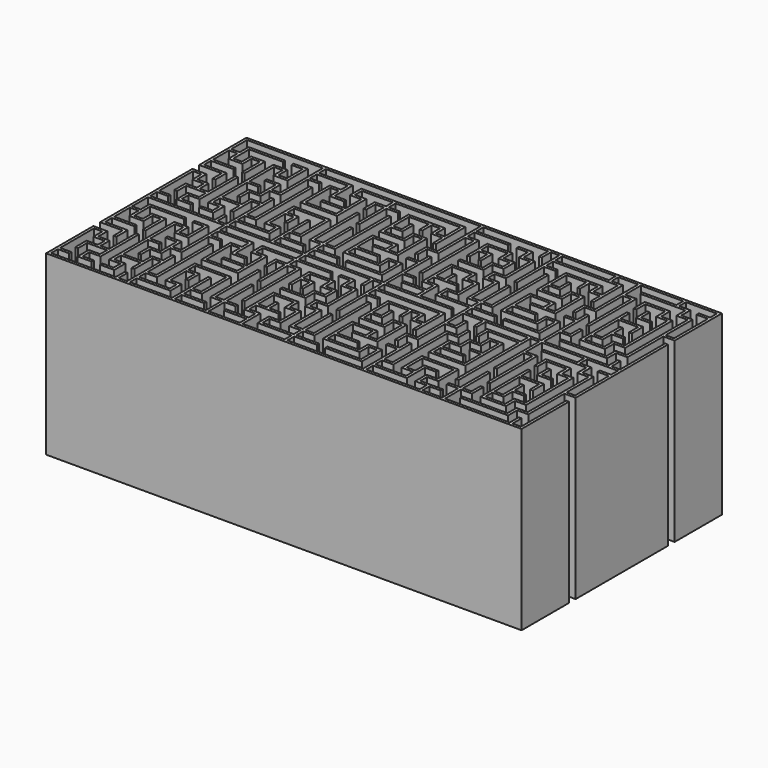
from build123d import *

# Parameters (mm, degrees)
F0_W     = 1.5875
F0_H     = 0.396875
F0_W_2   = 4.7625
F1_DEPTH = 25
F0_W_3   = 0.396875
F0_H_2   = 1.5875
F0_W_4   = 3.175
F0_H_3   = 7.9375
F0_W_5   = 10.715625


# Not quite as in the source:
# - a feature of the source that left no trace in its solid (it failed there, or was rolled back) is left out


with BuildPart() as f1:
    # F0 (on Top) → F1 (new body)
    with BuildSketch(Plane.XY):
        Polygon((-25.598351, 8.135938), (-25.598351, 6.151563), (-25.201476, 6.151563), (-25.201476, 7.739063), (-23.613976, 7.739063), (-23.613976, 9.326563), (-22.423351, 9.326563), (-22.423351, 9.723438), (-23.613976, 9.723438), (-23.613976, 11.310938), (-25.598351, 11.310938), (-25.598351, 10.914063), (-24.010851, 10.914063), (-24.010851, 8.135938), align=None)
        Polygon((-22.423351, 9.723438), (-22.423351, 9.326563), (-22.026476, 9.326563), (-22.026476, 14.089063), (-22.026476, 14.485938), (-22.026476, 15.676563), (-22.026476, 16.073438), (-22.026476, 17.264063), (-22.026476, 17.660938), (-22.423351, 17.660938), (-22.423351, 17.264063), align=None)
        with Locations((-21.232726, 14.2875005)):
            Rectangle(F0_W, F0_H)
        Polygon((-33.138976, 17.264063), (-22.423351, 17.264063), (-22.423351, 17.660938), (-33.535851, 17.660938), (-33.535851, 9.326563), (-30.360851, 9.326563), (-30.360851, 7.739063), (-29.963976, 7.739063), (-29.963976, 9.723438), (-33.138976, 9.723438), (-33.138976, 10.914063), (-29.963976, 10.914063), (-29.963976, 11.310938), (-33.138976, 11.310938), (-33.138976, 14.089063), (-31.948351, 14.089063), (-31.948351, 12.501563), (-29.963976, 12.501563), (-29.963976, 14.089063), (-28.773351, 14.089063), (-28.773351, 10.914063), (-28.376476, 10.914063), (-28.376476, 14.485938), (-30.360851, 14.485938), (-30.360851, 12.898438), (-31.551476, 12.898438), (-31.551476, 15.676563), (-26.788976, 15.676563), (-26.788976, 16.073438), (-31.948351, 16.073438), (-31.948351, 14.485938), (-33.138976, 14.485938), align=None)
        Polygon((-22.026476, 16.073438), (-22.026476, 15.676563), (-17.660851, 15.676563), (-17.660851, 14.485938), (-19.248351, 14.485938), (-19.248351, 9.326563), (-14.088976, 9.326563), (-14.088976, 14.485938), (-15.676476, 14.485938), (-15.676476, 15.676563), (-11.310851, 15.676563), (-11.310851, 14.485938), (-12.898351, 14.485938), (-12.898351, 12.501563), (-12.501476, 12.501563), (-12.501476, 14.089063), (-11.310851, 14.089063), (-11.310851, 9.326563), (-10.913976, 9.326563), (-10.913976, 14.089063), (-9.326476, 14.089063), (-9.326476, 14.485938), (-10.913976, 14.485938), (-10.913976, 15.676563), (-1.786023, 15.676563), (-1.786023, 12.898438), (-2.976648, 12.898438), (-2.976648, 14.485938), (-8.135851, 14.485938), (-8.135851, 9.326563), (-4.564148, 9.326563), (-4.564148, 10.914063), (-3.373523, 10.914063), (-3.373523, 6.548438), (-4.564148, 6.548438), (-4.564148, 8.135938), (-8.135851, 8.135938), (-8.135851, 2.976563), (-2.976648, 2.976563), (-2.976648, 4.564063), (-1.786023, 4.564063), (-1.786023, 1.785938), (-6.548351, 1.785938), (-6.548351, 1.389063), (-1.389148, 1.389063), (-1.389148, 4.960938), (-3.373523, 4.960938), (-3.373523, 3.373438), (-7.738976, 3.373438), (-7.738976, 4.564063), (-4.564148, 4.564063), (-4.564148, 4.960938), (-7.738976, 4.960938), (-7.738976, 7.739063), (-4.961023, 7.739063), (-4.961023, 6.548438), (-6.548351, 6.548438), (-6.548351, 6.151563), (-2.976648, 6.151563), (-2.976648, 11.310938), (-4.961023, 11.310938), (-4.961023, 9.723438), (-7.738976, 9.723438), (-7.738976, 10.914063), (-6.151476, 10.914063), (-6.151476, 12.898438), (-6.548351, 12.898438), (-6.548351, 11.310938), (-7.738976, 11.310938), (-7.738976, 14.089063), (-4.961023, 14.089063), (-4.961023, 12.501563), (-4.564148, 12.501563), (-4.564148, 14.089063), (-3.373523, 14.089063), (-3.373523, 12.501563), (-1.786023, 12.501563), (-1.786023, 10.914063), (-1.389148, 10.914063), (-1.389148, 16.073438), (-2.976648, 16.073438), (-3.373523, 16.073438), (-10.913976, 16.073438), (-11.310851, 16.073438), (-16.073351, 16.073438), (-16.073351, 14.089063), (-14.485851, 14.089063), (-14.485851, 11.310938), (-17.660851, 11.310938), (-17.660851, 10.914063), (-14.485851, 10.914063), (-14.485851, 9.723438), (-18.851476, 9.723438), (-18.851476, 14.089063), (-17.660851, 14.089063), (-17.660851, 12.501563), (-15.676476, 12.501563), (-15.676476, 12.898438), (-17.263976, 12.898438), (-17.263976, 16.073438), align=None)
        Polygon((-11.310851, 17.660938), (-22.026476, 17.660938), (-22.026476, 17.264063), (-11.310851, 17.264063), (-10.913976, 17.264063), (-3.373523, 17.264063), (-2.976648, 17.264063), (-0.198523, 17.264063), (-0.198523, 9.723438), (-0.198523, 9.326563), (0.198352, 9.326563), (0.198352, 14.089063), (0.198352, 14.485938), (0.198352, 15.676563), (0.198352, 16.073438), (0.198352, 17.264063), (9.326477, 17.264063), (9.326477, 15.676563), (9.723352, 15.676563), (9.723352, 17.264063), (10.913977, 17.264063), (10.913977, 17.660938), (0.198352, 17.660938), (-0.198523, 17.660938), (-10.913976, 17.660938), align=None)
        Polygon((11.310852, 17.660938), (10.913977, 17.660938), (10.913977, 17.264063), (10.913977, 9.326563), (11.310852, 9.326563), (11.310852, 14.089063), (11.310852, 14.485938), (11.310852, 15.676563), (11.310852, 16.073438), (11.310852, 17.264063), align=None)
        Polygon((22.026477, 17.660938), (11.310852, 17.660938), (11.310852, 17.264063), (18.851477, 17.264063), (18.851477, 16.073438), (11.310852, 16.073438), (11.310852, 15.676563), (20.438977, 15.676563), (20.438977, 12.898438), (19.248352, 12.898438), (19.248352, 14.485938), (14.088977, 14.485938), (14.088977, 9.326563), (17.660852, 9.326563), (17.660852, 10.914063), (18.851477, 10.914063), (18.851477, 6.548438), (17.660852, 6.548438), (17.660852, 8.135938), (14.088977, 8.135938), (14.088977, 2.976563), (19.248352, 2.976563), (19.248352, 4.564063), (20.438977, 4.564063), (20.438977, 1.785938), (15.676477, 1.785938), (15.676477, 1.389063), (20.835852, 1.389063), (20.835852, 4.960938), (18.851477, 4.960938), (18.851477, 3.373438), (14.485852, 3.373438), (14.485852, 4.564063), (17.660852, 4.564063), (17.660852, 4.960938), (14.485852, 4.960938), (14.485852, 7.739063), (17.263977, 7.739063), (17.263977, 6.548438), (15.676477, 6.548438), (15.676477, 6.151563), (19.248352, 6.151563), (19.248352, 11.310938), (17.263977, 11.310938), (17.263977, 9.723438), (14.485852, 9.723438), (14.485852, 10.914063), (16.073352, 10.914063), (16.073352, 12.898438), (15.676477, 12.898438), (15.676477, 11.310938), (14.485852, 11.310938), (14.485852, 14.089063), (17.263977, 14.089063), (17.263977, 12.501563), (17.660852, 12.501563), (17.660852, 14.089063), (18.851477, 14.089063), (18.851477, 12.501563), (20.438977, 12.501563), (20.438977, 10.914063), (20.835852, 10.914063), (20.835852, 16.073438), (19.248352, 16.073438), (19.248352, 17.264063), (22.026477, 17.264063), align=None)
        Polygon((-0.198523, 9.326563), (-0.198523, 9.723438), (-1.786023, 9.723438), (-1.786023, 7.739063), (-1.389148, 7.739063), (-1.389148, 9.326563), align=None)
        Polygon((22.423352, 17.660938), (22.026477, 17.660938), (22.026477, 17.264063), (22.026477, 9.723438), (22.026477, 9.326563), (22.423352, 9.326563), (22.423352, 14.089063), (22.423352, 14.485938), (22.423352, 17.264063), align=None)
        Polygon((33.535852, 17.660938), (22.423352, 17.660938), (22.423352, 17.264063), (28.376477, 17.264063), (28.376477, 16.073438), (23.613977, 16.073438), (23.613977, 15.676563), (29.963977, 15.676563), (29.963977, 14.089063), (31.551477, 14.089063), (31.551477, 3.373438), (29.963977, 3.373438), (29.963977, 1.785938), (23.613977, 1.785938), (23.613977, 1.389063), (30.360852, 1.389063), (30.360852, 2.976563), (31.948352, 2.976563), (31.948352, 9.326563), (33.535852, 9.326563), align=None)
        Polygon((33.138977, 15.676563), (33.138977, 9.723438), (31.948352, 9.723438), (31.948352, 14.485938), (30.360852, 14.485938), (30.360852, 16.073438), (28.773352, 16.073438), (28.773352, 17.264063), (33.138977, 17.264063), (33.138977, 16.073438), (31.551477, 16.073438), (31.551477, 15.676563), align=None, mode=Mode.SUBTRACT)
        Polygon((22.026477, 9.326563), (22.026477, 9.723438), (20.438977, 9.723438), (20.438977, 7.739063), (20.835852, 7.739063), (20.835852, 9.326563), align=None)
        with Locations((12.104602, 14.2875005)):
            Rectangle(F0_W, F0_H)
        Polygon((0.198352, 14.485938), (0.198352, 14.089063), (1.388977, 14.089063), (1.388977, 4.564063), (1.785852, 4.564063), (1.785852, 14.485938), align=None)
        Polygon((24.010852, 14.485938), (22.423352, 14.485938), (22.423352, 14.089063), (23.613977, 14.089063), (23.613977, 6.151563), (24.010852, 6.151563), align=None)
        with Locations((2.579602, 15.8750005)):
            Rectangle(F0_W_2, F0_H)
    extrude(amount=F1_DEPTH)


with BuildPart() as f1b:
    # F0 (on Top) → F1, piece 2 (new body)
    with BuildSketch(Plane.XY):
        Polygon((-33.535851, 0.198438), (-33.535851, -0.198437), (-33.138976, -0.198437), (-22.423351, -0.198437), (-22.423351, 0.198438), (-23.613976, 0.198438), (-24.010851, 0.198438), (-33.138976, 0.198438), align=None)
        Polygon((-33.138976, -0.198437), (-33.535851, -0.198437), (-33.535851, -8.135937), (-30.360851, -8.135937), (-30.360851, -9.723437), (-29.963976, -9.723437), (-29.963976, -7.739062), (-33.138976, -7.739062), (-33.138976, -6.548437), (-29.963976, -6.548437), (-29.963976, -6.151562), (-33.138976, -6.151562), (-33.138976, -3.373437), (-31.948351, -3.373437), (-31.948351, -4.960937), (-29.963976, -4.960937), (-29.963976, -3.373437), (-28.773351, -3.373437), (-28.773351, -6.548437), (-28.376476, -6.548437), (-28.376476, -2.976562), (-30.360851, -2.976562), (-30.360851, -4.564062), (-31.551476, -4.564062), (-31.551476, -1.785937), (-26.788976, -1.785937), (-26.788976, -1.389062), (-31.948351, -1.389062), (-31.948351, -2.976562), (-33.138976, -2.976562), align=None)
        Polygon((-33.535851, 8.135938), (-33.535851, 0.198438), (-33.138976, 0.198438), (-33.138976, 1.389063), (-31.551476, 1.389063), (-31.551476, 1.785938), (-33.138976, 1.785938), (-33.138976, 7.739063), (-31.948351, 7.739063), (-31.948351, 6.151563), (-30.360851, 6.151563), (-30.360851, 4.960938), (-31.948351, 4.960938), (-31.948351, 2.976563), (-31.551476, 2.976563), (-31.551476, 4.564063), (-28.773351, 4.564063), (-28.773351, 3.373438), (-30.360851, 3.373438), (-30.360851, 1.389063), (-28.376476, 1.389063), (-28.376476, 1.785938), (-29.963976, 1.785938), (-29.963976, 2.976563), (-28.376476, 2.976563), (-28.376476, 9.723438), (-28.773351, 9.723438), (-28.773351, 4.960938), (-29.963976, 4.960938), (-29.963976, 6.548438), (-31.551476, 6.548438), (-31.551476, 8.135938), align=None)
        with Locations((-22.2249135, 5e-07)):
            Rectangle(F0_W_3, F0_H)
        Polygon((-22.026476, -0.198437), (-22.423351, -0.198437), (-22.423351, -7.739062), (-22.423351, -8.135937), (-22.026476, -8.135937), (-22.026476, -3.373437), (-22.026476, -2.976562), (-22.026476, -1.785937), (-22.026476, -1.389062), align=None)
        with Locations((-23.8124135, 0.992188)):
            Rectangle(F0_W_3, F0_H_2)
        Polygon((-22.026476, 0.198438), (-22.026476, -0.198437), (-11.310851, -0.198437), (-11.310851, 0.198438), (-15.676476, 0.198438), (-16.073351, 0.198438), align=None)
        Polygon((-22.423351, 6.151563), (-22.423351, 0.198438), (-22.026476, 0.198438), (-22.026476, 1.389063), (-22.026476, 1.785938), (-22.026476, 2.976563), (-22.026476, 3.373438), (-22.026476, 8.135938), (-22.423351, 8.135938), (-22.423351, 6.548438), align=None)
        Polygon((-22.423351, -8.135937), (-22.423351, -7.739062), (-23.613976, -7.739062), (-23.613976, -6.151562), (-25.598351, -6.151562), (-25.598351, -6.548437), (-24.010851, -6.548437), (-24.010851, -9.326562), (-25.598351, -9.326562), (-25.598351, -11.310937), (-25.201476, -11.310937), (-25.201476, -9.723437), (-23.613976, -9.723437), (-23.613976, -8.135937), align=None)
        with Locations((-11.1124135, 5e-07)):
            Rectangle(F0_W_3, F0_H)
        Polygon((-10.913976, -0.198437), (-11.310851, -0.198437), (-11.310851, -1.389062), (-11.310851, -1.785937), (-11.310851, -2.976562), (-11.310851, -3.373437), (-11.310851, -8.135937), (-10.913976, -8.135937), (-10.913976, -3.373437), (-10.913976, -2.976562), (-10.913976, -1.785937), (-10.913976, -1.389062), align=None)
        Polygon((-17.263976, -1.389062), (-22.026476, -1.389062), (-22.026476, -1.785937), (-17.660851, -1.785937), (-17.660851, -2.976562), (-19.248351, -2.976562), (-19.248351, -8.135937), (-14.088976, -8.135937), (-14.088976, -2.976562), (-15.676476, -2.976562), (-15.676476, -1.785937), (-11.310851, -1.785937), (-11.310851, -1.389062), (-16.073351, -1.389062), (-16.073351, -3.373437), (-14.485851, -3.373437), (-14.485851, -6.151562), (-17.660851, -6.151562), (-17.660851, -6.548437), (-14.485851, -6.548437), (-14.485851, -7.739062), (-18.851476, -7.739062), (-18.851476, -3.373437), (-17.660851, -3.373437), (-17.660851, -4.960937), (-15.676476, -4.960937), (-15.676476, -4.564062), (-17.263976, -4.564062), align=None)
        Polygon((-23.613976, 6.151563), (-22.423351, 6.151563), (-22.423351, 6.548438), (-24.010851, 6.548438), (-24.010851, 4.960938), (-26.788976, 4.960938), (-26.788976, 9.326563), (-25.201476, 9.326563), (-25.201476, 9.723438), (-26.788976, 9.723438), (-26.788976, 14.089063), (-25.598351, 14.089063), (-25.598351, 12.501563), (-23.613976, 12.501563), (-23.613976, 16.073438), (-25.598351, 16.073438), (-25.598351, 15.676563), (-24.010851, 15.676563), (-24.010851, 12.898438), (-25.201476, 12.898438), (-25.201476, 14.485938), (-27.185851, 14.485938), (-27.185851, 2.976563), (-25.598351, 2.976563), (-25.598351, 1.785938), (-27.185851, 1.785938), (-27.185851, 1.389063), (-25.201476, 1.389063), (-25.201476, 3.373438), (-26.788976, 3.373438), (-26.788976, 4.564063), (-24.010851, 4.564063), (-24.010851, 2.976563), (-23.613976, 2.976563), align=None)
        Polygon((-22.026476, 1.785938), (-22.026476, 1.389063), (-17.263976, 1.389063), (-17.263976, 3.373438), (-18.851476, 3.373438), (-18.851476, 6.151563), (-17.660851, 6.151563), (-17.660851, 4.564063), (-17.263976, 4.564063), (-17.263976, 6.548438), (-18.851476, 6.548438), (-18.851476, 7.739063), (-14.485851, 7.739063), (-14.485851, 3.373438), (-15.676476, 3.373438), (-15.676476, 6.548438), (-16.073351, 6.548438), (-16.073351, 0.198438), (-15.676476, 0.198438), (-15.676476, 1.389063), (-12.501476, 1.389063), (-12.501476, 1.785938), (-15.676476, 1.785938), (-15.676476, 2.976563), (-14.088976, 2.976563), (-14.088976, 8.135938), (-19.248351, 8.135938), (-19.248351, 2.976563), (-17.660851, 2.976563), (-17.660851, 1.785938), align=None)
        Polygon((-10.913976, 0.198438), (-10.913976, -0.198437), (-1.786023, -0.198437), (-1.389148, -0.198437), (-0.198523, -0.198437), (-0.198523, 0.198438), align=None)
        Polygon((-11.310851, 2.976563), (-11.310851, 0.198438), (-10.913976, 0.198438), (-10.913976, 1.389063), (-10.913976, 1.785938), (-10.913976, 2.976563), (-10.913976, 3.373438), (-10.913976, 8.135938), (-11.310851, 8.135938), (-11.310851, 3.373438), align=None)
        with Locations((-1.5875855, -0.992187)):
            Rectangle(F0_W_3, F0_H_2)
        with Locations((-8.532726, -1.5874995)):
            Rectangle(F0_W_2, F0_H)
        Polygon((-12.898351, 2.976563), (-11.310851, 2.976563), (-11.310851, 3.373438), (-12.501476, 3.373438), (-12.501476, 11.310938), (-12.898351, 11.310938), align=None)
        with Locations((-21.232726, -3.1749995)):
            Rectangle(F0_W, F0_H)
        Polygon((-22.026476, 3.373438), (-22.026476, 2.976563), (-20.438976, 2.976563), (-20.438976, 12.898438), (-20.835851, 12.898438), (-20.835851, 3.373438), align=None)
        with Locations((-9.326476, 1.5875005)):
            Rectangle(F0_W_4, F0_H)
        with Locations((-8.55e-05, 5e-07)):
            Rectangle(F0_W_3, F0_H)
        Polygon((-0.198523, 6.151563), (-0.198523, 0.198438), (0.198352, 0.198438), (0.198352, 2.976563), (0.198352, 3.373438), (0.198352, 8.135938), (-0.198523, 8.135938), (-0.198523, 6.548438), align=None)
        Polygon((-11.310851, -3.373437), (-11.310851, -2.976562), (-12.898351, -2.976562), (-12.898351, -4.960937), (-12.501476, -4.960937), (-12.501476, -3.373437), align=None)
        with Locations((-0.992273, 6.3500005)):
            Rectangle(F0_W, F0_H)
        Polygon((0.198352, -0.198437), (-0.198523, -0.198437), (-0.198523, -8.135937), (0.198352, -8.135937), (0.198352, -3.373437), (0.198352, -2.976562), (0.198352, -1.785937), (0.198352, -1.389062), align=None)
        Polygon((4.563977, 0.198438), (0.198352, 0.198438), (0.198352, -0.198437), (7.738977, -0.198437), (8.135852, -0.198437), (9.6680196002, -0.198437), (9.6819251776, -0.198437), (9.6680196002, 0.198438), (4.960852, 0.198438), align=None)
        Polygon((-9.326476, -2.976562), (-10.913976, -2.976562), (-10.913976, -3.373437), (-9.723351, -3.373437), (-9.723351, -12.898437), (-9.326476, -12.898437), align=None)
        Polygon((-10.913976, 3.373438), (-10.913976, 2.976563), (-9.326476, 2.976563), (-9.326476, 12.898438), (-9.723351, 12.898438), (-9.723351, 3.373438), align=None)
        with Locations((0.992102, 3.1750005)):
            Rectangle(F0_W, F0_H)
        Polygon((4.563977, 1.389063), (4.563977, 0.198438), (4.960852, 0.198438), (4.960852, 3.373438), (3.373352, 3.373438), (3.373352, 4.564063), (6.548352, 4.564063), (6.548352, 4.960938), (4.960852, 4.960938), (4.960852, 6.548438), (4.563977, 6.548438), (4.563977, 4.960938), (3.373352, 4.960938), (3.373352, 7.739063), (6.151477, 7.739063), (6.151477, 6.151563), (7.738977, 6.151563), (7.738977, 3.373438), (6.151477, 3.373438), (6.151477, 1.389063), (10.913977, 1.389063), (10.913977, 1.785938), (6.548352, 1.785938), (6.548352, 2.976563), (8.135852, 2.976563), (8.135852, 6.548438), (6.548352, 6.548438), (6.548352, 8.135938), (2.976477, 8.135938), (2.976477, 2.976563), (4.563977, 2.976563), (4.563977, 1.785938), (1.388977, 1.785938), (1.388977, 1.389063), align=None)
        Polygon((7.738977, -1.389062), (0.198352, -1.389062), (0.198352, -1.785937), (9.326477, -1.785937), (9.326477, -4.564062), (8.135852, -4.564062), (8.135852, -2.976562), (2.976477, -2.976562), (2.976477, -8.135937), (6.548352, -8.135937), (6.548352, -6.548437), (7.738977, -6.548437), (7.738977, -10.914062), (6.548352, -10.914062), (6.548352, -9.326562), (2.976477, -9.326562), (2.976477, -14.485937), (8.135852, -14.485937), (8.135852, -12.898437), (9.326477, -12.898437), (9.326477, -15.676562), (4.563977, -15.676562), (4.563977, -16.073437), (9.723352, -16.073437), (9.723352, -12.501562), (7.738977, -12.501562), (7.738977, -14.089062), (3.373352, -14.089062), (3.373352, -12.898437), (6.548352, -12.898437), (6.548352, -12.501562), (3.373352, -12.501562), (3.373352, -9.723437), (6.151477, -9.723437), (6.151477, -10.914062), (4.563977, -10.914062), (4.563977, -11.310937), (8.135852, -11.310937), (8.135852, -6.151562), (6.151477, -6.151562), (6.151477, -7.739062), (3.373352, -7.739062), (3.373352, -6.548437), (4.960852, -6.548437), (4.960852, -4.564062), (4.563977, -4.564062), (4.563977, -6.151562), (3.373352, -6.151562), (3.373352, -3.373437), (6.151477, -3.373437), (6.151477, -4.960937), (6.548352, -4.960937), (6.548352, -3.373437), (7.738977, -3.373437), (7.738977, -4.960937), (9.326477, -4.960937), (9.326477, -6.548437), (9.723352, -6.548437), (9.723352, -1.389062), (8.135977, -1.389062), (8.135852, -1.389062), align=None)
        with Locations((0.992102, -3.1749995)):
            Rectangle(F0_W, F0_H)
        Polygon((10.913977, 2.976563), (10.913977, 1.785938), (10.913977, 1.389063), (10.913977, 0.198438), (11.310852, 0.198438), (11.310852, 1.389063), (11.310852, 1.785938), (11.310852, 2.976563), (11.310852, 3.373438), (11.310852, 8.135938), (10.913977, 8.135938), (10.913977, 3.373438), align=None)
        Polygon((9.326477, 2.976563), (10.913977, 2.976563), (10.913977, 3.373438), (9.723352, 3.373438), (9.723352, 8.135938), (8.135852, 8.135938), (8.135852, 9.326563), (9.723352, 9.326563), (9.723352, 14.485938), (8.135852, 14.485938), (8.135852, 16.073438), (6.151477, 16.073438), (6.151477, 15.676563), (7.738977, 15.676563), (7.738977, 14.089063), (9.326477, 14.089063), (9.326477, 9.723438), (7.738977, 9.723438), (7.738977, 7.739063), (9.326477, 7.739063), align=None)
        with Locations((11.1124145, 5e-07)):
            Rectangle(F0_W_3, F0_H)
        Polygon((11.310852, -0.198437), (10.913977, -0.198437), (10.913977, -7.739062), (10.913977, -8.135937), (11.310852, -8.135937), (11.310852, -3.373437), (11.310852, -2.976562), align=None)
        Polygon((22.026477, 0.198438), (11.310852, 0.198438), (11.310852, -0.198437), (14.088977, -0.198437), (14.485852, -0.198437), (20.438977, -0.198437), (20.835852, -0.198437), (22.026477, -0.198437), align=None)
        Polygon((10.913977, -8.135937), (10.913977, -7.739062), (9.326477, -7.739062), (9.326477, -9.723437), (9.723352, -9.723437), (9.723352, -8.135937), align=None)
        with Locations((12.898352, 1.5875005)):
            Rectangle(F0_W_4, F0_H)
        with Locations((22.2249145, 5e-07)):
            Rectangle(F0_W_3, F0_H)
        Polygon((22.026477, 6.151563), (22.026477, 0.198438), (22.423352, 0.198438), (22.423352, 2.976563), (22.423352, 3.373438), (22.423352, 8.135938), (22.026477, 8.135938), (22.026477, 6.548438), align=None)
        Polygon((12.501477, 3.373438), (11.310852, 3.373438), (11.310852, 2.976563), (12.898352, 2.976563), (12.898352, 12.898438), (12.501477, 12.898438), align=None)
        with Locations((14.2874145, -0.992187)):
            Rectangle(F0_W_3, F0_H_2)
        Polygon((12.501477, -2.976562), (11.310852, -2.976562), (11.310852, -3.373437), (12.898352, -3.373437), (12.898352, -1.389062), (12.501477, -1.389062), align=None)
        with Locations((21.232727, 6.3500005)):
            Rectangle(F0_W, F0_H)
        Polygon((22.423352, -0.198437), (22.026477, -0.198437), (22.026477, -8.135937), (22.423352, -8.135937), (22.423352, -3.373437), (22.423352, -2.976562), align=None)
        Polygon((31.551477, 0.198438), (22.423352, 0.198438), (22.423352, -0.198437), (28.376477, -0.198437), (28.773352, -0.198437), (33.138977, -0.198437), (33.535852, -0.198437), (33.535852, 0.198438), (33.138977, 0.198438), (31.948352, 0.198438), align=None)
        Polygon((20.835852, -12.898437), (20.835852, -0.198437), (20.438977, -0.198437), (20.438977, -1.389062), (15.676477, -1.389062), (15.676477, -3.373437), (16.073352, -3.373437), (16.073352, -1.785937), (20.438977, -1.785937), (20.438977, -12.898437), align=None)
        Polygon((22.423352, 3.373438), (22.423352, 2.976563), (24.010852, 2.976563), (24.010852, 4.960938), (23.613977, 4.960938), (23.613977, 3.373438), align=None)
        with Locations((31.7499145, 0.992188)):
            Rectangle(F0_W_3, F0_H_2)
        Polygon((28.773352, -0.198437), (28.376477, -0.198437), (28.376477, -1.389062), (23.613977, -1.389062), (23.613977, -1.785937), (29.963977, -1.785937), (29.963977, -3.373437), (31.551477, -3.373437), (31.551477, -14.089062), (29.963977, -14.089062), (29.963977, -15.676562), (23.613977, -15.676562), (23.613977, -16.073437), (30.360852, -16.073437), (30.360852, -14.485937), (31.948352, -14.485937), (31.948352, -8.135937), (33.535852, -8.135937), (33.535852, -0.198437), (33.138977, -0.198437), (33.138977, -1.389062), (31.551477, -1.389062), (31.551477, -1.785937), (33.138977, -1.785937), (33.138977, -7.739062), (31.948352, -7.739062), (31.948352, -2.976562), (30.360852, -2.976562), (30.360852, -1.389062), (28.773352, -1.389062), align=None)
        Polygon((24.010852, -2.976562), (22.423352, -2.976562), (22.423352, -3.373437), (23.613977, -3.373437), (23.613977, -11.310937), (24.010852, -11.310937), align=None)
        with Locations((33.3374145, 4.167188)):
            Rectangle(F0_W_3, F0_H_3)
    extrude(amount=F1_DEPTH)


with BuildPart() as f1c:
    # F0 (on Top) → F1, piece 3 (new body)
    with BuildSketch(Plane.XY):
        Polygon((2.976477, 9.723438), (2.976477, 9.326563), (6.548352, 9.326563), (6.548352, 10.914063), (8.135852, 10.914063), (8.135852, 12.898438), (6.548352, 12.898438), (6.548352, 14.485938), (2.976477, 14.485938), (2.976477, 10.914063), (3.373352, 10.914063), (3.373352, 12.501563), (4.563977, 12.501563), (4.563977, 10.914063), (4.960852, 10.914063), (4.960852, 12.898438), (3.373352, 12.898438), (3.373352, 14.089063), (6.151477, 14.089063), (6.151477, 12.501563), (7.738977, 12.501563), (7.738977, 11.310938), (6.151477, 11.310938), (6.151477, 9.723438), align=None)
    extrude(amount=F1_DEPTH)


with BuildPart() as f1d:
    # F0 (on Top) → F1, piece 4 (new body)
    with BuildSketch(Plane.XY):
        Polygon((25.201477, 11.310938), (25.201477, 2.976563), (28.773352, 2.976563), (28.773352, 4.564063), (30.360852, 4.564063), (30.360852, 12.898438), (28.773352, 12.898438), (28.773352, 14.485938), (25.201477, 14.485938), (25.201477, 12.501563), (25.598352, 12.501563), (25.598352, 14.089063), (28.376477, 14.089063), (28.376477, 12.501563), (29.963977, 12.501563), (29.963977, 4.960938), (28.376477, 4.960938), (28.376477, 3.373438), (25.598352, 3.373438), (25.598352, 4.564063), (27.185852, 4.564063), (27.185852, 6.151563), (28.773352, 6.151563), (28.773352, 6.548438), (27.185852, 6.548438), (27.185852, 8.135938), (26.788977, 8.135938), (26.788977, 4.960938), (25.598352, 4.960938), (25.598352, 9.326563), (28.376477, 9.326563), (28.376477, 7.739063), (28.773352, 7.739063), (28.773352, 9.723438), (25.598352, 9.723438), (25.598352, 11.310938), align=None)
    extrude(amount=F1_DEPTH)


with BuildPart() as f1e:
    # F0 (on Top) → F1, piece 5 (new body)
    with BuildSketch(Plane.XY):
        Polygon((26.788977, 12.898438), (26.788977, 10.914063), (28.773352, 10.914063), (28.773352, 11.310938), (27.185852, 11.310938), (27.185852, 12.898438), align=None)
    extrude(amount=F1_DEPTH)


with BuildPart() as f1f:
    # F0 (on Top) → F1, piece 6 (new body)
    with BuildSketch(Plane.XY):
        Polygon((-33.535851, -9.326562), (-33.535851, -17.660937), (-22.423351, -17.660937), (-22.423351, -17.264062), (-23.613976, -17.264062), (-23.613976, -15.676562), (-24.010851, -15.676562), (-24.010851, -17.264062), (-33.138976, -17.264062), (-33.138976, -16.073437), (-31.551476, -16.073437), (-31.551476, -15.676562), (-33.138976, -15.676562), (-33.138976, -9.723437), (-31.948351, -9.723437), (-31.948351, -11.310937), (-30.360851, -11.310937), (-30.360851, -12.501562), (-31.948351, -12.501562), (-31.948351, -14.485937), (-31.551476, -14.485937), (-31.551476, -12.898437), (-28.773351, -12.898437), (-28.773351, -14.089062), (-30.360851, -14.089062), (-30.360851, -16.073437), (-28.376476, -16.073437), (-28.376476, -15.676562), (-29.963976, -15.676562), (-29.963976, -14.485937), (-28.376476, -14.485937), (-28.376476, -7.739062), (-28.773351, -7.739062), (-28.773351, -12.501562), (-29.963976, -12.501562), (-29.963976, -10.914062), (-31.551476, -10.914062), (-31.551476, -9.326562), align=None)
        Polygon((-22.423351, -17.264062), (-22.423351, -17.660937), (-22.026476, -17.660937), (-22.026476, -17.264062), (-22.026476, -16.073437), (-22.026476, -15.676562), (-22.026476, -14.485937), (-22.026476, -14.089062), (-22.026476, -9.326562), (-22.423351, -9.326562), (-22.423351, -10.914062), (-22.423351, -11.310937), align=None)
        Polygon((-22.026476, -17.264062), (-22.026476, -17.660937), (-11.310851, -17.660937), (-11.310851, -17.264062), (-15.676476, -17.264062), (-15.676476, -16.073437), (-12.501476, -16.073437), (-12.501476, -15.676562), (-15.676476, -15.676562), (-15.676476, -14.485937), (-14.088976, -14.485937), (-14.088976, -9.326562), (-19.248351, -9.326562), (-19.248351, -14.485937), (-17.660851, -14.485937), (-17.660851, -15.676562), (-22.026476, -15.676562), (-22.026476, -16.073437), (-17.263976, -16.073437), (-17.263976, -14.089062), (-18.851476, -14.089062), (-18.851476, -11.310937), (-17.660851, -11.310937), (-17.660851, -12.898437), (-17.263976, -12.898437), (-17.263976, -10.914062), (-18.851476, -10.914062), (-18.851476, -9.723437), (-14.485851, -9.723437), (-14.485851, -14.089062), (-15.676476, -14.089062), (-15.676476, -10.914062), (-16.073351, -10.914062), (-16.073351, -17.264062), align=None)
        Polygon((-11.310851, -17.264062), (-11.310851, -17.660937), (-10.913976, -17.660937), (-10.913976, -17.264062), (-10.913976, -14.485937), (-10.913976, -14.089062), (-10.913976, -9.326562), (-11.310851, -9.326562), (-11.310851, -14.089062), (-11.310851, -14.485937), align=None)
        Polygon((-23.613976, -11.310937), (-22.423351, -11.310937), (-22.423351, -10.914062), (-24.010851, -10.914062), (-24.010851, -12.501562), (-26.788976, -12.501562), (-26.788976, -8.135937), (-25.201476, -8.135937), (-25.201476, -7.739062), (-26.788976, -7.739062), (-26.788976, -3.373437), (-25.598351, -3.373437), (-25.598351, -4.960937), (-23.613976, -4.960937), (-23.613976, -1.389062), (-25.598351, -1.389062), (-25.598351, -1.785937), (-24.010851, -1.785937), (-24.010851, -4.564062), (-25.201476, -4.564062), (-25.201476, -2.976562), (-27.185851, -2.976562), (-27.185851, -14.485937), (-25.598351, -14.485937), (-25.598351, -15.676562), (-27.185851, -15.676562), (-27.185851, -16.073437), (-25.201476, -16.073437), (-25.201476, -14.089062), (-26.788976, -14.089062), (-26.788976, -12.898437), (-24.010851, -12.898437), (-24.010851, -14.485937), (-23.613976, -14.485937), align=None)
        Polygon((-10.913976, -17.264062), (-10.913976, -17.660937), (-0.198523, -17.660937), (-0.198523, -17.264062), (-6.151476, -17.264062), (-6.151476, -14.089062), (-7.738976, -14.089062), (-7.738976, -12.898437), (-4.564148, -12.898437), (-4.564148, -12.501562), (-6.151476, -12.501562), (-6.151476, -10.914062), (-6.548351, -10.914062), (-6.548351, -12.501562), (-7.738976, -12.501562), (-7.738976, -9.723437), (-4.961023, -9.723437), (-4.961023, -11.310937), (-3.373523, -11.310937), (-3.373523, -14.089062), (-4.961023, -14.089062), (-4.961023, -16.073437), (-0.198523, -16.073437), (-0.198523, -15.676562), (-4.564148, -15.676562), (-4.564148, -14.485937), (-2.976648, -14.485937), (-2.976648, -10.914062), (-4.564148, -10.914062), (-4.564148, -9.326562), (-8.135851, -9.326562), (-8.135851, -14.485937), (-6.548351, -14.485937), (-6.548351, -15.676562), (-9.723351, -15.676562), (-9.723351, -16.073437), (-6.548351, -16.073437), (-6.548351, -17.264062), align=None)
        Polygon((-0.198523, -17.264062), (-0.198523, -17.660937), (0.198352, -17.660937), (0.198352, -17.264062), (0.198352, -16.073437), (0.198352, -15.676562), (0.198352, -14.485937), (0.198352, -14.089062), (0.198352, -9.326562), (-0.198523, -9.326562), (-0.198523, -14.089062), (-0.198523, -14.485937), (-0.198523, -15.676562), (-0.198523, -16.073437), align=None)
        Polygon((-12.898351, -14.485937), (-11.310851, -14.485937), (-11.310851, -14.089062), (-12.501476, -14.089062), (-12.501476, -6.151562), (-12.898351, -6.151562), align=None)
        Polygon((-22.026476, -14.089062), (-22.026476, -14.485937), (-20.438976, -14.485937), (-20.438976, -4.564062), (-20.835851, -4.564062), (-20.835851, -14.089062), align=None)
        with Locations((-10.120226, -14.2874995)):
            Rectangle(F0_W, F0_H)
        with Locations((5.5561645, -17.4624995)):
            Rectangle(F0_W_5, F0_H)
        Polygon((10.913977, -17.264062), (10.913977, -17.660937), (11.310852, -17.660937), (11.310852, -17.264062), (11.310852, -16.073437), (11.310852, -15.676562), (11.310852, -14.485937), (11.310852, -14.089062), (11.310852, -9.326562), (10.913977, -9.326562), (10.913977, -10.914062), (10.913977, -11.310937), align=None)
        with Locations((1.785852, -15.8749995)):
            Rectangle(F0_W_4, F0_H)
        Polygon((11.310852, -17.264062), (11.310852, -17.660937), (22.026477, -17.660937), (22.026477, -17.264062), (19.248352, -17.264062), (19.248352, -16.073437), (20.835852, -16.073437), (20.835852, -15.676562), (17.660852, -15.676562), (17.660852, -14.485937), (19.248352, -14.485937), (19.248352, -10.914062), (14.088977, -10.914062), (14.088977, -14.485937), (15.676477, -14.485937), (15.676477, -15.676562), (11.310852, -15.676562), (11.310852, -16.073437), (16.073352, -16.073437), (16.073352, -12.898437), (17.660852, -12.898437), (17.660852, -12.501562), (15.676477, -12.501562), (15.676477, -14.089062), (14.485852, -14.089062), (14.485852, -11.310937), (18.851477, -11.310937), (18.851477, -14.089062), (17.263977, -14.089062), (17.263977, -16.073437), (18.851477, -16.073437), (18.851477, -17.264062), align=None)
        with Locations((10.120227, -11.1124995)):
            Rectangle(F0_W, F0_H)
        Polygon((22.026477, -17.264062), (22.026477, -17.660937), (22.423352, -17.660937), (22.423352, -17.264062), (22.423352, -14.485937), (22.423352, -14.089062), (22.423352, -9.723437), (22.026477, -9.723437), (22.026477, -14.089062), (22.026477, -14.485937), align=None)
        Polygon((-1.786023, -14.485937), (-0.198523, -14.485937), (-0.198523, -14.089062), (-1.389148, -14.089062), (-1.389148, -9.326562), (-2.976648, -9.326562), (-2.976648, -8.135937), (-1.389148, -8.135937), (-1.389148, -2.976562), (-2.976648, -2.976562), (-2.976648, -1.389062), (-4.961023, -1.389062), (-4.961023, -1.785937), (-3.373523, -1.785937), (-3.373523, -3.373437), (-1.786023, -3.373437), (-1.786023, -7.739062), (-3.373523, -7.739062), (-3.373523, -9.723437), (-1.786023, -9.723437), align=None)
        Polygon((0.198352, -14.089062), (0.198352, -14.485937), (1.785852, -14.485937), (1.785852, -4.564062), (1.388977, -4.564062), (1.388977, -14.089062), align=None)
        Polygon((22.423352, -17.264062), (22.423352, -17.660937), (33.535852, -17.660937), (33.535852, -9.326562), (33.138977, -9.326562), (33.138977, -17.264062), (31.948352, -17.264062), (31.948352, -15.676562), (31.551477, -15.676562), (31.551477, -17.264062), align=None)
        with Locations((21.232727, -14.2874995)):
            Rectangle(F0_W, F0_H)
        Polygon((11.310852, -14.089062), (11.310852, -14.485937), (12.898352, -14.485937), (12.898352, -4.960937), (14.485852, -4.960937), (14.485852, -2.976562), (14.088977, -2.976562), (14.088977, -4.564062), (12.501477, -4.564062), (12.501477, -14.089062), align=None)
        Polygon((22.423352, -14.089062), (22.423352, -14.485937), (24.010852, -14.485937), (24.010852, -12.501562), (23.613977, -12.501562), (23.613977, -14.089062), align=None)
        with Locations((22.2249145, -9.5249995)):
            Rectangle(F0_W_3, F0_H)
    extrude(amount=F1_DEPTH)


with BuildPart() as f1g:
    # F0 (on Top) → F1, piece 7 (new body)
    with BuildSketch(Plane.XY):
        Polygon((-8.135851, -7.739062), (-8.135851, -8.135937), (-4.564148, -8.135937), (-4.564148, -6.548437), (-2.976648, -6.548437), (-2.976648, -4.564062), (-4.564148, -4.564062), (-4.564148, -2.976562), (-8.135851, -2.976562), (-8.135851, -6.548437), (-7.738976, -6.548437), (-7.738976, -4.960937), (-6.548351, -4.960937), (-6.548351, -6.548437), (-6.151476, -6.548437), (-6.151476, -4.564062), (-7.738976, -4.564062), (-7.738976, -3.373437), (-4.961023, -3.373437), (-4.961023, -4.960937), (-3.373523, -4.960937), (-3.373523, -6.151562), (-4.961023, -6.151562), (-4.961023, -7.739062), align=None)
    extrude(amount=F1_DEPTH)


with BuildPart() as f1h:
    # F0 (on Top) → F1, piece 8 (new body)
    with BuildSketch(Plane.XY):
        Polygon((14.088977, -6.151562), (14.088977, -9.723437), (19.248352, -9.723437), (19.248352, -2.976562), (17.263977, -2.976562), (17.263977, -4.564062), (15.676477, -4.564062), (15.676477, -6.151562), align=None)
        Polygon((18.851477, -6.548437), (18.851477, -9.326562), (14.485852, -9.326562), (14.485852, -8.135937), (17.660852, -8.135937), (17.660852, -7.739062), (14.485852, -7.739062), (14.485852, -6.548437), (16.073352, -6.548437), (16.073352, -4.960937), (17.660852, -4.960937), (17.660852, -3.373437), (18.851477, -3.373437), (18.851477, -6.151562), (17.263977, -6.151562), (17.263977, -6.548437), align=None, mode=Mode.SUBTRACT)
    extrude(amount=F1_DEPTH)


with BuildPart() as f1i:
    # F0 (on Top) → F1, piece 9 (new body)
    with BuildSketch(Plane.XY):
        Polygon((25.201477, -6.151562), (25.201477, -14.485937), (28.773352, -14.485937), (28.773352, -12.898437), (30.360852, -12.898437), (30.360852, -4.564062), (28.773352, -4.564062), (28.773352, -2.976562), (25.201477, -2.976562), (25.201477, -4.960937), (25.598352, -4.960937), (25.598352, -3.373437), (28.376477, -3.373437), (28.376477, -4.960937), (29.963977, -4.960937), (29.963977, -12.501562), (28.376477, -12.501562), (28.376477, -14.089062), (25.598352, -14.089062), (25.598352, -12.898437), (27.185852, -12.898437), (27.185852, -11.310937), (28.773352, -11.310937), (28.773352, -10.914062), (27.185852, -10.914062), (27.185852, -9.326562), (26.788977, -9.326562), (26.788977, -12.501562), (25.598352, -12.501562), (25.598352, -8.135937), (28.376477, -8.135937), (28.376477, -9.723437), (28.773352, -9.723437), (28.773352, -7.739062), (25.598352, -7.739062), (25.598352, -6.151562), align=None)
    extrude(amount=F1_DEPTH)


with BuildPart() as f1j:
    # F0 (on Top) → F1, piece 10 (new body)
    with BuildSketch(Plane.XY):
        Polygon((26.788977, -4.564062), (26.788977, -6.548437), (28.773352, -6.548437), (28.773352, -6.151562), (27.185852, -6.151562), (27.185852, -4.564062), align=None)
    extrude(amount=F1_DEPTH)


solid = Compound([f1.part, f1b.part, f1c.part, f1d.part, f1e.part, f1f.part, f1g.part, f1h.part, f1i.part, f1j.part])
